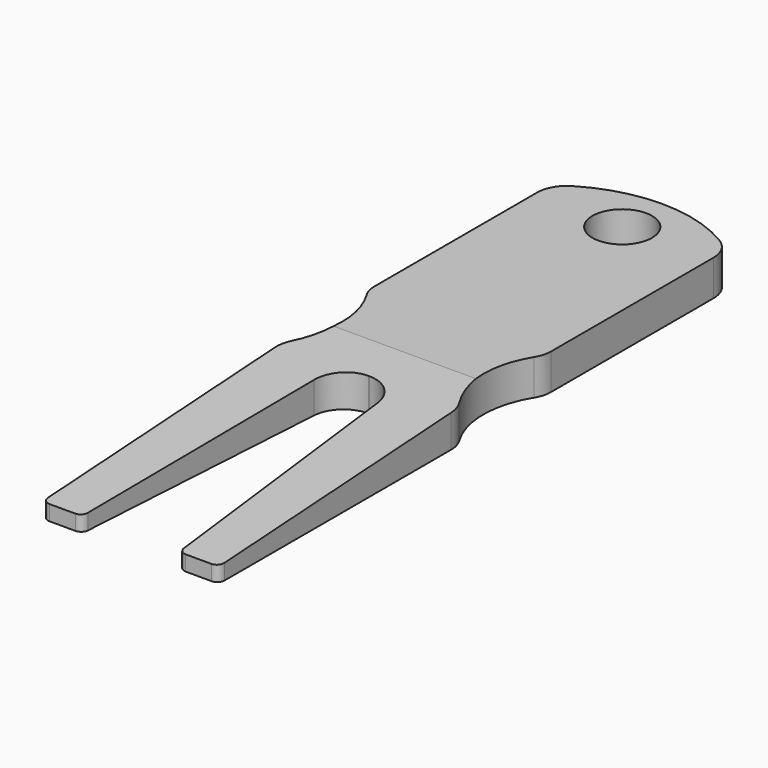
from build123d import *

# Parameters (mm, degrees)
F0_R        = 3.175
F1_DEPTH    = 3.81
F2_R        = 3.302
F3_T1_DEPTH = 7.6195000328
F3_T3_DEPTH = 7.3891966687
F5_DEPTH    = 3.811
F6_R        = 3.175
F8_DEPTH    = 18.797


# Not quite as in the source:
# - a fillet or chamfer that OpenCascade refuses, or shapes differently, is made with other operations: its cross-section is extruded or revolved along the edge and cut away or added


with BuildPart() as f1:
    # F0 (on Top) → F1 (new body)
    with BuildSketch(Plane.XY):
        with BuildLine():
            ThreePointArc((8.9284270597, -22.9513050998), (7.6006411438, -16.7271260659), (10.4890512239, -11.0561025874))
            ThreePointArc((10.4890512239, -11.0561025874), (0, 15.24), (-10.4890512239, -11.0561025874))
            ThreePointArc((-10.4890512239, -11.0561025874), (-7.6006411438, -16.7271260659), (-8.9284270597, -22.9513050998))
            ThreePointArc((-8.9284270597, -22.9513050998), (-9.2783523459, -23.7496251472), (-9.398, -24.6130178983))
            Line((-9.398, -24.6130178983), (-9.398, -55.5625))
            Line((-9.398, -55.5625), (-5.1562, -55.5625))
            Line((-5.1562, -55.5625), (-3.175, -23.8125))
            Line((-3.175, -23.8125), (3.175, -23.8125))
            Line((3.175, -23.8125), (5.1562, -55.5625))
            Line((5.1562, -55.5625), (9.398, -55.5625))
            Line((9.398, -55.5625), (9.398, -24.6130178983))
            ThreePointArc((9.398, -24.6130178983), (9.2783523459, -23.7496251472), (8.9284270597, -22.9513050998))
        make_face()
        with Locations((0, 9.921875)):
            Circle(F0_R, mode=Mode.SUBTRACT)
    extrude(amount=-F1_DEPTH)

    # F2
    f2_edges = [f1.edges().sort_by_distance(p)[0] for p in [
        (-3.175, -23.8125, -1.905),
        (3.175, -23.8125, -1.905),
    ]]
    fillet(f2_edges, radius=F2_R)

    # F3: fillet of radius 0.762 on 4 edges, made by hand

    # F3_s2 → F3_t1 (cut)
    with BuildSketch(Plane.XY.offset(-5.7147500164)):
        with BuildLine():
            ThreePointArc((8.6361, -55.5626), (9.1749153673, -55.3394153673), (9.3981, -54.8006))
            Line((9.3981, -54.8006), (9.41334, -54.8006))
            ThreePointArc((9.41334, -54.8006), (9.41324, -55.18155), (9.41324, -55.5625))
            Line((9.41324, -55.5625), (9.398, -55.57774))
            ThreePointArc((9.398, -55.57774), (9.01705, -55.57774), (8.6361, -55.57784))
            Line((8.6361, -55.57784), (8.6361, -55.5626))
        make_face()
        with BuildLine():
            ThreePointArc((-8.6361, -55.5626), (-9.1749153673, -55.3394153673), (-9.3981, -54.8006))
            Line((-9.3981, -54.8006), (-9.41334, -54.8006))
            ThreePointArc((-9.41334, -54.8006), (-9.41324, -55.18155), (-9.41324, -55.5625))
            Line((-9.41324, -55.5625), (-9.398, -55.57774))
            ThreePointArc((-9.398, -55.57774), (-9.01705, -55.57774), (-8.6361, -55.57784))
            Line((-8.6361, -55.57784), (-8.6361, -55.5626))
        make_face()
    extrude(amount=F3_T1_DEPTH, mode=Mode.SUBTRACT)

    # F3_s4 → F3_t3 (cut)
    with BuildSketch(Plane.XY.offset(-5.5995983343)):
        with BuildLine():
            ThreePointArc((-5.111518531, -54.8480564977), (-5.350272066, -55.3559403691), (-5.8720393267, -55.5626))
            Line((-5.8720393267, -55.5626), (-5.8720393267, -55.57784))
            ThreePointArc((-5.8720393267, -55.57784), (-5.5141196634, -55.57774), (-5.1562, -55.57774))
            Line((-5.1562, -55.57774), (-5.1409895841, -55.56344913))
            ThreePointArc((-5.1409895841, -55.56344913), (-5.1186987525, -55.2062242648), (-5.096308115, -54.8490056276))
            Line((-5.096308115, -54.8490056276), (-5.111518531, -54.8480564977))
        make_face()
        with BuildLine():
            ThreePointArc((5.111518531, -54.8480564977), (5.350272066, -55.3559403691), (5.8720393267, -55.5626))
            Line((5.8720393267, -55.5626), (5.8720393267, -55.57784))
            ThreePointArc((5.8720393267, -55.57784), (5.5141196634, -55.57774), (5.1562, -55.57774))
            Line((5.1562, -55.57774), (5.1409895841, -55.56344913))
            ThreePointArc((5.1409895841, -55.56344913), (5.1186987525, -55.2062242648), (5.096308115, -54.8490056276))
            Line((5.096308115, -54.8490056276), (5.111518531, -54.8480564977))
        make_face()
    extrude(amount=F3_T3_DEPTH, mode=Mode.SUBTRACT)

    # F4 (on face) → F5 (cut, through all)
    with BuildSketch(Plane.XY):
        Polygon((-9.398, -15.875), (-9.398, 17.78), (9.398, 17.78), (9.398, -15.875), (19.05, -15.875), (19.05, 20.32), (-19.05, 20.32), (-19.05, -15.875), align=None)
    extrude(amount=-F5_DEPTH, mode=Mode.SUBTRACT)

    # F6
    f6_edges = [f1.edges().sort_by_distance(p)[0] for p in [
        (9.398, 11.9973, -1.905),
        (-9.398, 11.9973, -1.905),
        (-9.398, -12.286952, -1.905),
        (9.398, -12.286952, -1.905),
    ]]
    fillet(f6_edges, radius=F6_R)

    # F7 (on face) → F8 (cut, through all)
    with BuildSketch(Plane.YZ.offset(9.398)):
        Polygon((-57.15, 0), (-57.15, -2.286), (-19.05, 0), align=None)
    extrude(amount=-F8_DEPTH, mode=Mode.SUBTRACT)


solid = f1.part
